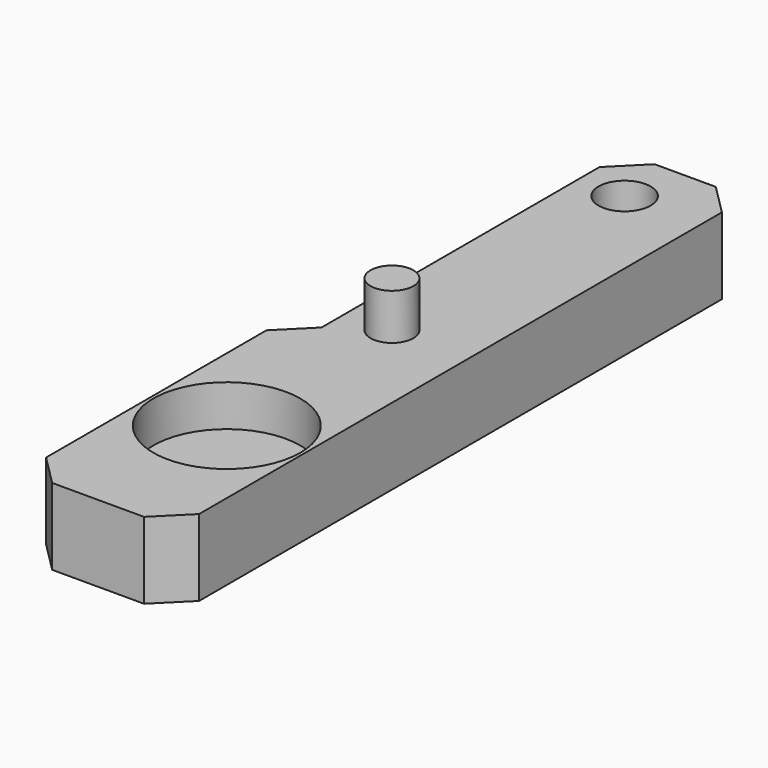
from build123d import *

# Parameters (mm, degrees)
F0_W     = 8
F0_H     = 26.7
F0_R     = 1.4
F0_R_2   = 1.7
F0_R_3   = 4.8
F1_DEPTH = 5
F2_DEPTH = 8
F0_R_4   = 2.8
F3_DEPTH = 2.3
F4_START = 2
F4_DEPTH = 0.3
F5_SIZE  = 1.99999


# Not quite as in the source:
# - a fillet or chamfer is up to 0.001 mm smaller than in the source, because OpenCascade refuses the exact size


with BuildPart() as f1:
    # F0 (on Top) → F1 (new body)
    with BuildSketch(Plane.XY):
        with Locations((1, 4.0926239572)):
            Rectangle(F0_W, F0_H)
        with Locations((0, -5.2573760428)):
            Circle(F0_R, mode=Mode.SUBTRACT)
        with Locations((0, 13.7426239572)):
            Circle(F0_R_2, mode=Mode.SUBTRACT)
        Polygon((-5, -9.2573760428), (-5, -29.2573760428), (5, -29.2573760428), (5, -9.2573760428), (-3, -9.2573760428), align=None)
        with Locations((0, -18.7472271925)):
            Circle(F0_R_3, mode=Mode.SUBTRACT)
    extrude(amount=F1_DEPTH)

    # F0 (on Top) → F2 (join)
    with BuildSketch(Plane.XY):
        with Locations((0, -5.2573760428)):
            Circle(F0_R)
    extrude(amount=F2_DEPTH)

    # F0 (on Top) → F3 (join)
    with BuildSketch(Plane.XY):
        with Locations((0, -18.7472271925)):
            Circle(F0_R_3)
        with Locations((0, -18.7472271925)):
            Circle(F0_R_4, mode=Mode.SUBTRACT)
    extrude(amount=F3_DEPTH)

    # F0 (on Top) → F4 (join)
    with BuildSketch(Plane.XY.offset(F4_START)):
        with Locations((0, -18.7472271925)):
            Circle(F0_R_4)
    extrude(amount=F4_DEPTH)

    # F5 (size 2 in the source; OpenCascade refuses exactly that, so slightly less here)
    f5_edges = [f1.edges().sort_by_distance(p)[0] for p in [
        (-3, -9.257376, 2.5),
        (-3, 17.442624, 2.5),
        (5, 17.442624, 2.5),
        (5, -29.257376, 2.5),
        (-5, -29.257376, 2.5),
    ]]
    chamfer(f5_edges, length=F5_SIZE)


solid = f1.part
